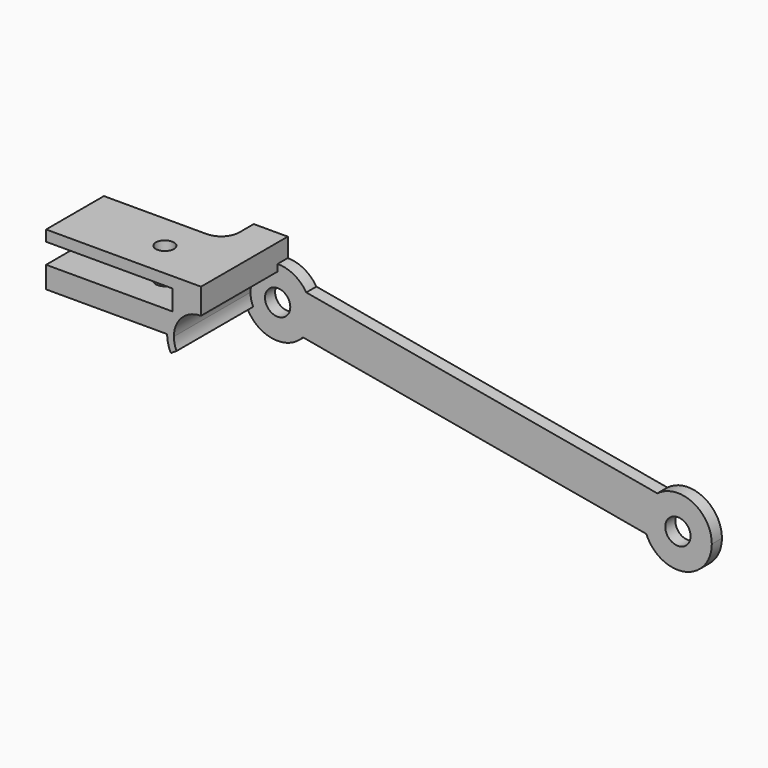
from build123d import *

# Parameters (mm, degrees)
F0_R      = 1.778
F1_DEPTH  = 17.78
F3_R      = 1.778
F4_DEPTH  = 16.002
F2_R      = 1.27
F5_DEPTH  = 25.4
F7_DEPTH  = 2.54
F8_W      = 16.9942029752
F8_H      = 1.524
F8_H_2    = 3.048
F9_DEPTH  = 5.08
F11_DEPTH = 13.462
F12_R     = 2.54


# Not quite as in the source:
# - a feature names something its author has since deleted; it is built from what else it names


with BuildPart() as f1:
    # F0 (on Front) → F1 (new body)
    with BuildSketch(Plane.XZ):
        with BuildLine():
            Line((-21.7745867558, 0), (-5.7350052521, 0))
            Line((-5.7350052521, 0), (-4.7625, 0))
            ThreePointArc((-4.7625, 0), (-3.3675960454, 3.3675960454), (0, 4.7625))
            Line((0, 4.7625), (0, 7.4168))
            Line((0, 7.4168), (-21.7745867558, 7.4168))
            Line((-21.7745867558, 7.4168), (-21.7745867558, 5.8928))
            Line((-21.7745867558, 5.8928), (-3.9945867558, 5.8928))
            Line((-3.9945867558, 5.8928), (-3.9945867558, 3.048))
            Line((-3.9945867558, 3.048), (-21.7745867558, 3.048))
            Line((-21.7745867558, 3.048), (-21.7745867558, 0))
        make_face()
        with BuildLine():
            ThreePointArc((4.7625, 0), (4.4508557537, -1.6944879196), (3.5567092138, -3.1672110474))
            Line((3.5567092138, -3.1672110474), (51.8252535905, -11.7928625561))
            ThreePointArc((51.8252535905, -11.7928625561), (51.6705317006, -8.7770103), (53.3605608921, -6.2743906673))
            Line((53.3605608921, -6.2743906673), (4.0277059432, 2.5414545216))
            ThreePointArc((4.0277059432, 2.5414545216), (4.5751150698, 1.3227729767), (4.7625, 0))
        make_face()
        with BuildLine():
            ThreePointArc((0, 4.7625), (-3.3675960454, 3.3675960454), (-4.7625, 0))
            ThreePointArc((-4.7625, 0), (-1.6944879196, -4.4508557537), (3.5567092138, -3.1672110474))
            ThreePointArc((3.5567092138, -3.1672110474), (4.4508557537, -1.6944879196), (4.7625, 0))
            ThreePointArc((4.7625, 0), (4.5751150698, 1.3227729767), (4.0277059432, 2.5414545216))
            ThreePointArc((4.0277059432, 2.5414545216), (2.2997531488, 4.1704366324), (0, 4.7625))
        make_face()
        Circle(F0_R, mode=Mode.SUBTRACT)
        with BuildLine():
            ThreePointArc((53.3605608921, -6.2743906673), (51.6705317006, -8.7770103), (51.8252535905, -11.7928625561))
            ThreePointArc((51.8252535905, -11.7928625561), (57.1438640566, -14.7330470759), (61.0212711223, -10.0535153956))
            ThreePointArc((61.0212711223, -10.0535153956), (58.3657452594, -5.7824422007), (53.3605608921, -6.2743906673))
        make_face()
        with Locations((56.2587711223, -10.0535153956)):
            Circle(F0_R, mode=Mode.SUBTRACT)
    extrude(amount=F1_DEPTH)

    # F3 (on face) → F4 (cut)
    with BuildSketch(Plane.XZ.offset(17.78)):
        with BuildLine():
            ThreePointArc((4.0277059432, 2.5414545216), (2.2997531488, 4.1704366324), (0, 4.7625))
            ThreePointArc((0, 4.7625), (-3.3675960454, 3.3675960454), (-4.7625, 0))
            ThreePointArc((-4.7625, 0), (-4.5665768899, -1.3519547915), (-3.994927608, -2.5926742288))
            ThreePointArc((-3.994927608, -2.5926742288), (-0.3612920968, -4.7487760813), (3.5567092138, -3.1672110474))
            Line((3.5567092138, -3.1672110474), (51.8252535905, -11.7928625561))
            ThreePointArc((51.8252535905, -11.7928625561), (60.847010544, -11.3300204911), (53.3605608921, -6.2743906673))
            Line((53.3605608921, -6.2743906673), (4.0277059432, 2.5414545216))
        make_face()
        with Locations((56.2587711223, -10.0535153956)):
            Circle(F3_R, mode=Mode.SUBTRACT)
        Circle(F3_R, mode=Mode.SUBTRACT)
    extrude(amount=-F4_DEPTH, mode=Mode.SUBTRACT)

    # F2 (on face) → F5 (cut)
    with BuildSketch(Plane.XY.offset(7.4168)):
        with Locations((-9.1804936528, -10.1120751351)):
            Circle(F2_R)
    extrude(amount=-F5_DEPTH, mode=Mode.SUBTRACT)

    # F6 (on face) → F7 (cut)
    with BuildSketch(Plane.XZ.offset(17.78)):
        with BuildLine():
            Line((-21.7745867558, 0), (-4.7625, 0))
            ThreePointArc((-4.7625, 0), (-3.3675960454, 3.3675960454), (0, 4.7625))
            Line((0, 4.7625), (0, 7.4168))
            Line((0, 7.4168), (-21.7745867558, 7.4168))
            Line((-21.7745867558, 7.4168), (-21.7745867558, 5.8928))
            Line((-21.7745867558, 5.8928), (-3.9945867558, 5.8928))
            Line((-3.9945867558, 5.8928), (-3.9945867558, 3.048))
            Line((-3.9945867558, 3.048), (-21.7745867558, 3.048))
            Line((-21.7745867558, 3.048), (-21.7745867558, 0))
        make_face()
    extrude(amount=-F7_DEPTH, mode=Mode.SUBTRACT)

    # F8 (on face) → F9 (cut)
    with BuildSketch(Plane(origin=(0, 0, 0), x_dir=(-1, 0, 0), z_dir=(0, 1, 0))):
        with Locations((13.2774852682, 6.6548)):
            Rectangle(F8_W, F8_H)
        with Locations((13.2774852682, 1.524)):
            Rectangle(F8_W, F8_H_2)
    extrude(amount=-F9_DEPTH, mode=Mode.SUBTRACT)

    # F10 (on face) → F11 (join, through all)
    with BuildSketch(Plane.XZ.offset(1.778)):
        with BuildLine():
            ThreePointArc((-3.8153238056, 0), (-2.6978413354, 2.6978413354), (0, 3.8153238056))
            Line((0, 3.8153238056), (0, 4.7625))
            ThreePointArc((0, 4.7625), (-3.3675960454, 3.3675960454), (-4.7625, 0))
            Line((-4.7625, 0), (-3.8153238056, 0))
        make_face()
        with BuildLine():
            Line((-4.2348116803, -2.1789392561), (-3.434889127, -1.6607927104))
            ThreePointArc((-3.434889127, -1.6607927104), (-3.7189991932, -0.8519041865), (-3.8153238056, 0))
            Line((-3.8153238056, 0), (-4.7625, 0))
            ThreePointArc((-4.7625, 0), (-4.6286983525, -1.1209628946), (-4.2348116803, -2.1789392561))
        make_face()
    extrude(amount=F11_DEPTH)

    # F12
    f12_edges = [f1.edges().sort_by_distance(p)[0] for p in [
        (-4.780384, -5.08, 1.524),
        (-4.780384, -5.08, 6.6548),
    ]]
    fillet(f12_edges, radius=F12_R)


solid = f1.part
